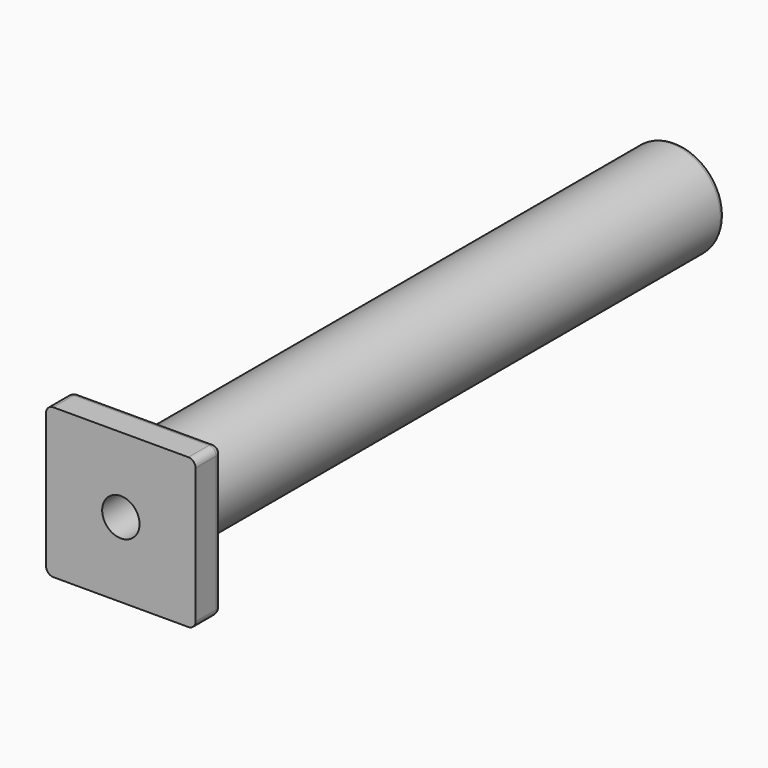
from build123d import *

# Parameters (mm, degrees)
F0_W     = 50.8
F0_H     = 50.8
F0_R     = 16.5908146865
F1_DEPTH = 11.176
F0_R_2   = 6.35
F2_DEPTH = 235.712
F3_R     = 2.4528409794
F4_R     = 2.4528409794
F5_R     = 2.4528409794
F6_R     = 2.4528409794
F7_R     = 1.8396307345


# Not quite as in the source:
# - a fillet or chamfer that OpenCascade refuses, or shapes differently, is made with other operations: its cross-section is extruded or revolved along the edge and cut away or added


with BuildPart() as f1:
    # F0 (on Front) → F1 (new body)
    with BuildSketch(Plane.XZ):
        Rectangle(F0_W, F0_H)
        Circle(F0_R, mode=Mode.SUBTRACT)
    extrude(amount=-F1_DEPTH)

    # F0 (on Front) → F2 (join)
    with BuildSketch(Plane.XZ):
        Circle(F0_R)
        Circle(F0_R_2, mode=Mode.SUBTRACT)
    extrude(amount=-F2_DEPTH)

    # F3
    f3_edges = [f1.edges().sort_by_distance(p)[0] for p in [
        (-25.4, 11.176, 0),
    ]]
    fillet(f3_edges, radius=F3_R)

    # F4
    f4_edges = [f1.edges().sort_by_distance(p)[0] for p in [
        (1.22642, 11.176, 25.4),
    ]]
    fillet(f4_edges, radius=F4_R)

    # F5
    f5_edges = [f1.edges().sort_by_distance(p)[0] for p in [
        (25.4, 11.176, -1.22642),
    ]]
    fillet(f5_edges, radius=F5_R)

    # F6
    f6_edges = [f1.edges().sort_by_distance(p)[0] for p in [
        (0, 11.176, -25.4),
    ]]
    fillet(f6_edges, radius=F6_R)

    # F7
    f7_edges = [f1.edges().sort_by_distance(p)[0] for p in [
        (-16.590815, 235.712, 0),
    ]]
    fillet(f7_edges, radius=F7_R)

    # F8: chamfer of 10.16 on 1 edges, made by hand

    # F8_s1 → F8_t2 (revolve, cut)
    with BuildSketch(Plane.XY):
        Polygon((16.51, 235.712), (6.35, 225.552), (6.35, 235.712), align=None)
    revolve(axis=Axis((0, 235.712, 0), (0, -1, 0)), mode=Mode.SUBTRACT)


solid = f1.part
